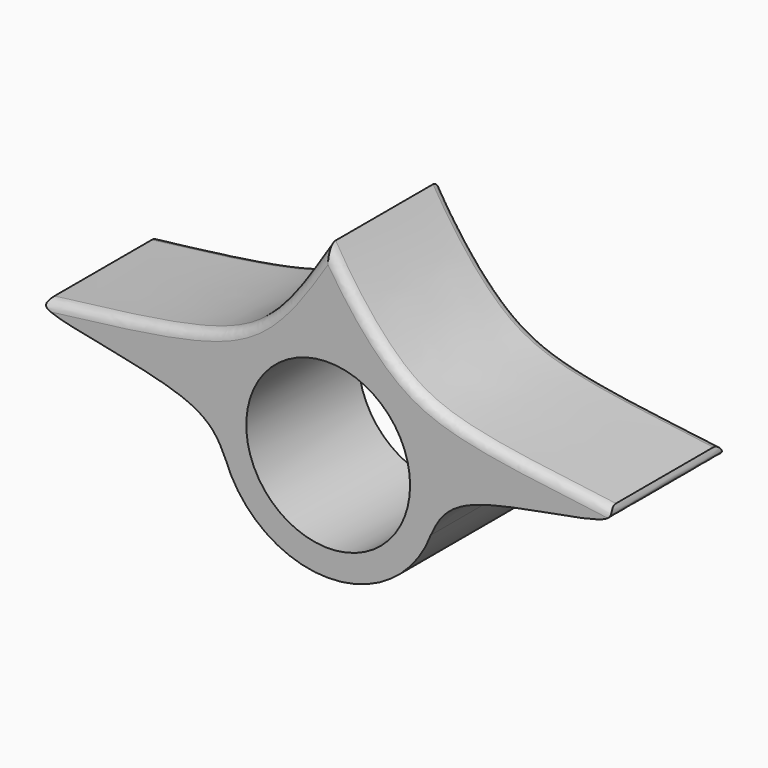
from build123d import *

# Parameters (mm, degrees)
F0_R     = 11.1155463884
F1_DEPTH = 19.05
F2_R     = 1.27


with BuildPart() as f1:
    # F0 (on Front) → F1 (new body)
    with BuildSketch(Plane.XZ):
        with BuildLine():
            add(Edge.make_bspline(
                [(-38.1638994336, 0), (-19.6957219024, 2.1979471251), (-9.311880126, 4.0390839853), (-2.7506002225, 14.761891216), (0, 19.05)],
                knots=[0, 0, 0, 0, 0.5912055263, 1, 1, 1, 1], degree=3))
            add(Edge.make_bspline(
                [(-13.9198412699, -11.1125), (-14.794313883, -9.2288451722), (-17.1100002201, -4.2407487086), (-39.5685055328, -1.9231498725), (-38.3696140076, -0.2816590053), (-38.1638994336, 0)],
                knots=[0, 0, 0, 0, 0.3345084593, 0.8858100955, 1, 1, 1, 1], degree=3))
            ThreePointArc((-13.9198412699, -11.1125), (0, -20.7508764), (13.9198412699, -11.1125))
            add(Edge.make_bspline(
                [(13.9198412699, -11.1125), (14.8240544816, -9.1946143672), (17.2053802942, -4.1436921907), (39.2933100068, -2.4877446669), (38.244207933, -0.4117993191), (38.0361005664, 0)],
                knots=[0, 0, 0, 0, 0.3291827069, 0.8669318993, 1, 1, 1, 1], degree=3))
            add(Edge.make_bspline(
                [(38.0361005664, 0), (20.2584086937, 2.241044324), (10.7040125651, 3.3870131368), (2.4307208404, 14.9494804331), (0, 19.05)],
                knots=[0, 0, 0, 0, 0.5801098598, 1, 1, 1, 1], degree=3))
        make_face()
        with Locations((0, -6.0836733319)):
            Circle(F0_R, mode=Mode.SUBTRACT)
    extrude(amount=F1_DEPTH)

    # F2
    f2_edges = [f1.edges().sort_by_distance(p)[0] for p in [
        (15.828231, -19.05, 3.702963),
        (15.828231, 0, 3.702963),
        (-15.834222, -19.05, 3.677027),
        (-15.834222, 0, 3.677027),
    ]]
    fillet(f2_edges, radius=F2_R)


solid = f1.part
